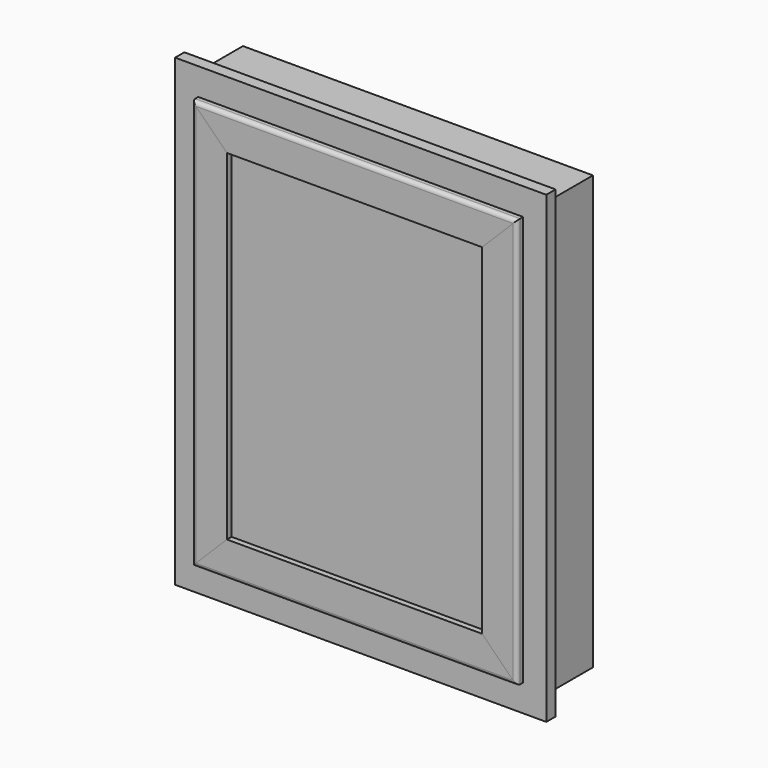
from build123d import *

# Parameters (mm, degrees)
F0_W      = 609.6
F0_H      = 762
F0_W_2    = 533.4
F0_H_2    = 673.1
F1_DEPTH  = 19.05
F2_W      = 574.675
F2_H      = 711.2
F2_W_2    = 533.4
F2_H_2    = 673.1
F3_DEPTH  = 98.425
F5_DEPTH  = 12.7
F6_DEPTH  = 12.7
F7_R      = 6.35
F7_2_R    = 6.35
F8_W      = 438.15
F8_H      = 19.05
F9_DEPTH  = 3.175
F10_W     = 19.05
F10_H     = 577.85
F11_DEPTH = 3.175
F14_W     = 434.975
F14_H     = 574.675
F15_DEPTH = 3.175
F16_W     = 530.225
F16_H     = 669.925
F17_DEPTH = 6.35
F18_W     = 527.05
F18_H     = 666.75
F19_DEPTH = 6.35


# Not quite as in the source:
# - a feature names something its author has since deleted; it is built from what else it names


with BuildPart() as f1:
    # F0 (on Front) → F1 (new body)
    with BuildSketch(Plane.XZ):
        Rectangle(F0_W, F0_H)
        Rectangle(F0_W_2, F0_H_2, mode=Mode.SUBTRACT)
    extrude(amount=F1_DEPTH)

    # F2 (on face) → F3 (join)
    with BuildSketch(Plane(origin=(0, 0, 0), x_dir=(-1, 0, 0), z_dir=(0, 1, 0))):
        Rectangle(F2_W, F2_H)
        Rectangle(F2_W_2, F2_H_2, mode=Mode.SUBTRACT)
    extrude(amount=F3_DEPTH)


with BuildPart() as f5:
    # F4 (on face) → F5 (new body)
    with BuildSketch(Plane.XZ.offset(19.05)):
        Polygon((209.55, 279.4), (266.7, 336.55), (-266.7, 336.55), (-209.55, 279.4), align=None)
    extrude(amount=F5_DEPTH)

    # F7
    f7_edges = [f5.edges().sort_by_distance(p)[0] for p in [
        (0, -31.75, 336.55),
    ]]
    fillet(f7_edges, radius=F7_R)


with BuildPart() as f6:
    # F4 (on face) → F6 (new body)
    with BuildSketch(Plane.XZ.offset(19.05)):
        Polygon((-209.55, 279.4), (-266.7, 336.55), (-266.7, -336.55), (-209.55, -279.4), align=None)
    extrude(amount=F6_DEPTH)

    # F7#2
    f7_2_edges = [f6.edges().sort_by_distance(p)[0] for p in [
        (-266.7, -31.75, 0),
    ]]
    fillet(f7_2_edges, radius=F7_2_R)


with BuildPart() as f9_tool:
    # F8 (on face) → F9 (new body)
    with BuildSketch(Plane(origin=(0, -19.05, 0), x_dir=(-1, 0, 0), z_dir=(0, 1, 0))):
        with Locations((0, 279.4)):
            Rectangle(F8_W, F8_H)
    extrude(amount=-F9_DEPTH)


with BuildPart() as f5_1:
    add(f5.part)

    # F9: cut by f9_tool
    add(f9_tool.part, mode=Mode.SUBTRACT)


with BuildPart() as f6_1:
    add(f6.part)

    # F9: cut by f9_tool
    add(f9_tool.part, mode=Mode.SUBTRACT)

    # F10 (on face) → F11 (cut)
    with BuildSketch(Plane(origin=(0, -19.05, 0), x_dir=(-1, 0, 0), z_dir=(0, 1, 0))):
        with Locations((209.55, 0)):
            Rectangle(F10_W, F10_H)
    extrude(amount=-F11_DEPTH, mode=Mode.SUBTRACT)


with BuildPart() as f12_1:
    # F12: instance of F6
    add(f6_1.part.mirror(Plane.YZ))


with BuildPart() as f13_1:
    # F13: instance of F5
    add(f5_1.part.mirror(Plane.XY))


with BuildPart() as f15:
    # F14 (on face) → F15 (new body)
    with BuildSketch(Plane(origin=(0, -22.225, 0), x_dir=(-1, 0, 0), z_dir=(0, 1, 0))):
        Rectangle(F14_W, F14_H)
    extrude(amount=F15_DEPTH)


with BuildPart() as f17:
    # F16 (on face) → F17 (new body)
    with BuildSketch(Plane(origin=(0, -19.05, 0), x_dir=(-1, 0, 0), z_dir=(0, 1, 0))):
        Rectangle(F16_W, F16_H)
    extrude(amount=F17_DEPTH)


with BuildPart() as f19:
    # F18 (on face) → F19 (new body)
    with BuildSketch(Plane(origin=(0, -19.05, 0), x_dir=(-1, 0, 0), z_dir=(0, 1, 0))):
        Rectangle(F18_W, F18_H)
    extrude(amount=F19_DEPTH)


solid = Compound([f1.part, f5_1.part, f6_1.part, f12_1.part, f13_1.part, f15.part, f19.part])
